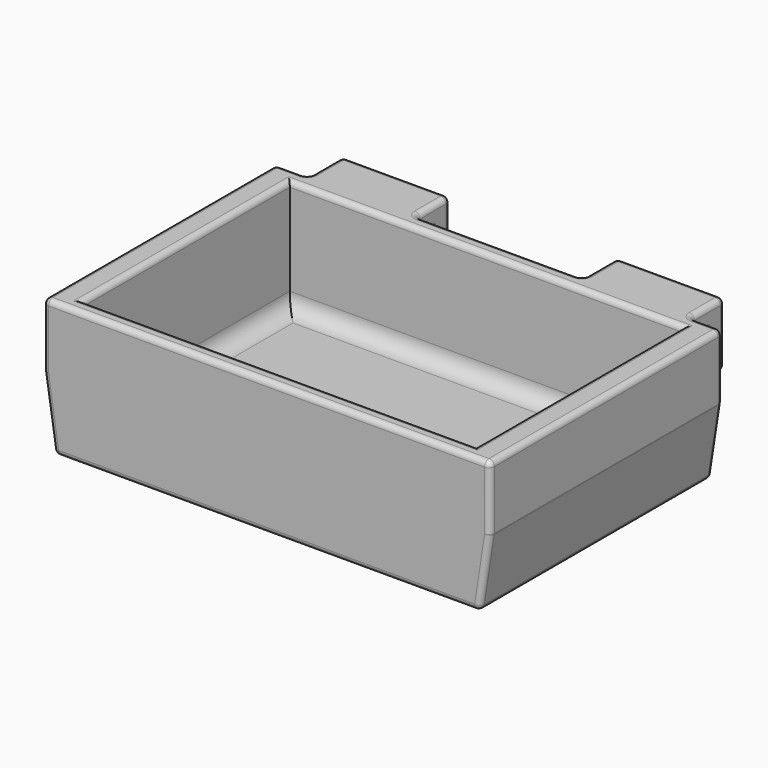
from build123d import *

# Parameters (mm, degrees)
F0_W     = 73
F0_H     = 48
F1_DEPTH = 4
F0_W_2   = 79
F0_H_2   = 54
F2_DEPTH = 25
F3_W     = 2
F3_H     = 12
F4_DEPTH = 54
F5_W     = 20
F5_H     = 12
F6_DEPTH = 8
F7_W     = 3.5
F7_H     = 8
F8_DEPTH = 80
F9_R     = 3
F10_R    = 1


with BuildPart() as f1:
    # F0 (on Top) → F1 (new body)
    with BuildSketch(Plane.XY):
        Rectangle(F0_W, F0_H)
    extrude(amount=F1_DEPTH)

    # F0 (on Top) → F2 (join)
    with BuildSketch(Plane.XY):
        Rectangle(F0_W_2, F0_H_2)
        Rectangle(F0_W, F0_H, mode=Mode.SUBTRACT)
    extrude(amount=F2_DEPTH)

    # F3 (on face) → F4 (join)
    with BuildSketch(Plane.XZ.offset(27)):
        with Locations((40.5, 19)):
            Rectangle(F3_W, F3_H)
        Polygon((39.5, 13), (39.5, 0), (41.5, 13), align=None)
        with Locations((-40.5, 19)):
            Rectangle(F3_W, F3_H)
        Polygon((-41.5, 13), (-39.5, 0), (-39.5, 13), align=None)
    extrude(amount=-F4_DEPTH)

    # F5 (on face) → F6 (join)
    with BuildSketch(Plane(origin=(0, 27, 0), x_dir=(-1, 0, 0), z_dir=(0, 1, 0))):
        with Locations((-25.5, 19)):
            Rectangle(F5_W, F5_H)
        with Locations((25.5, 19)):
            Rectangle(F5_W, F5_H)
    extrude(amount=F6_DEPTH)

    # F7 (on face) → F8 (cut)
    with BuildSketch(Plane(origin=(-35.5, 0, 0), x_dir=(0, -1, 0), z_dir=(-1, 0, 0))):
        with Locations((-28.75, 17)):
            Rectangle(F7_W, F7_H)
    extrude(amount=-F8_DEPTH, mode=Mode.SUBTRACT)

    # F9
    f9_edges = [f1.edges().sort_by_distance(p)[0] for p in [
        (0, -24, 4),
        (36.5, 0, 4),
        (0, 24, 4),
        (-36.5, 0, 4),
    ]]
    fillet(f9_edges, radius=F9_R)

    # F10
    f10_edges = [f1.edges().sort_by_distance(p)[0] for p in [
        (0, -27, 25),
        (41.5, 0, 25),
        (38.5, 27, 25),
        (35.5, 31, 25),
        (25.5, 35, 25),
        (15.5, 31, 25),
        (0, 27, 25),
        (-15.5, 31, 25),
        (-25.5, 35, 25),
        (-35.5, 31, 25),
        (-38.5, 27, 25),
        (-41.5, 0, 25),
        (36.5, 0, 25),
        (0, -24, 25),
        (-36.5, 0, 25),
        (0, 24, 25),
        (0, -27, 0),
        (39.5, 0, 0),
        (0, 27, 0),
        (-39.5, 0, 0),
        (-40.5, -27, 6.5),
        (-41.5, -27, 19),
        (41.5, -27, 19),
        (40.5, -27, 6.5),
        (41.5, 0, 13),
        (40.5, 27, 6.5),
        (41.5, 27, 19),
        (-41.5, 0, 13),
        (-40.5, 27, 6.5),
        (-41.5, 27, 19),
        (-15.5, 35, 19),
        (-25.5, 35, 13),
        (-35.5, 35, 19),
        (35.5, 35, 19),
        (25.5, 35, 13),
        (15.5, 35, 19),
        (25.5, 30.5, 13),
        (15.5, 32.75, 13),
        (35.5, 32.75, 13),
        (-25.5, 30.5, 13),
        (-35.5, 32.75, 13),
        (-15.5, 32.75, 13),
        (-15.5, 27, 23),
        (-15.5, 28.75, 21),
        (-15.5, 30.5, 17),
        (35.5, 27, 23),
        (35.5, 28.75, 21),
        (35.5, 30.5, 17),
        (15.5, 30.5, 17),
        (15.5, 28.75, 21),
        (15.5, 27, 23),
        (-35.5, 30.5, 17),
        (-35.5, 28.75, 21),
        (-35.5, 27, 23),
        (25.5, 27, 21),
        (-25.5, 27, 21),
    ]]
    fillet(f10_edges, radius=F10_R)


solid = f1.part
